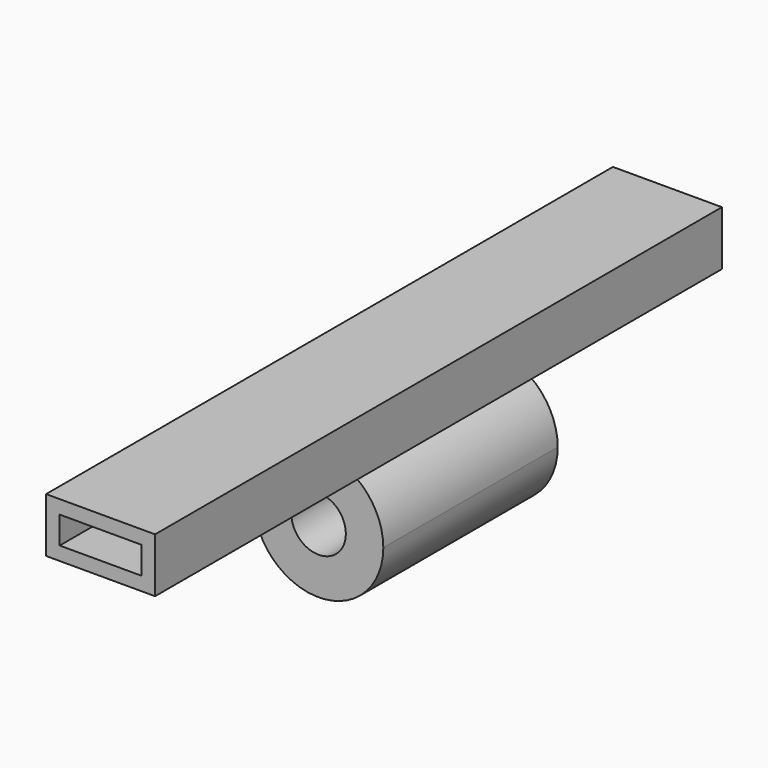
from build123d import *

# Parameters (mm, degrees)
F0_W     = 50.8
F0_H     = 25.4
F0_W_2   = 38.1
F0_H_2   = 12.7
F1_DEPTH = 330.2
F2_R     = 30.1625
F3_DEPTH = 228.6
F4_R     = 30.1625
F5_DEPTH = 127
F6_R     = 12.7
F7_DEPTH = 101.6


# Not quite as in the source:
# - a feature names something its author has since deleted; it is built from what else it names


with BuildPart() as f1:
    # F0 (on Front) → F1 (new body)
    with BuildSketch(Plane.XZ):
        with Locations((25.4, 12.7)):
            Rectangle(F0_W, F0_H)
        with Locations((25.4, 12.7)):
            Rectangle(F0_W_2, F0_H_2, mode=Mode.SUBTRACT)
    extrude(amount=F1_DEPTH)

    # F2 (on face) → F3 (join)
    with BuildSketch(Plane.XZ.offset(330.2)):
        with Locations((25.4, -30.1625)):
            Circle(F2_R)
    extrude(amount=-F3_DEPTH)

    # F4 (on face) → F5 (cut)
    with BuildSketch(Plane.XZ.offset(330.2)):
        with Locations((25.4, -30.1625)):
            Circle(F4_R)
    extrude(amount=-F5_DEPTH, mode=Mode.SUBTRACT)

    # F6 (on face) → F7 (cut, through all)
    with BuildSketch(Plane.XZ.offset(203.2)):
        with Locations((25.4, -30.1625)):
            Circle(F6_R)
    extrude(amount=-F7_DEPTH, mode=Mode.SUBTRACT)


solid = f1.part
